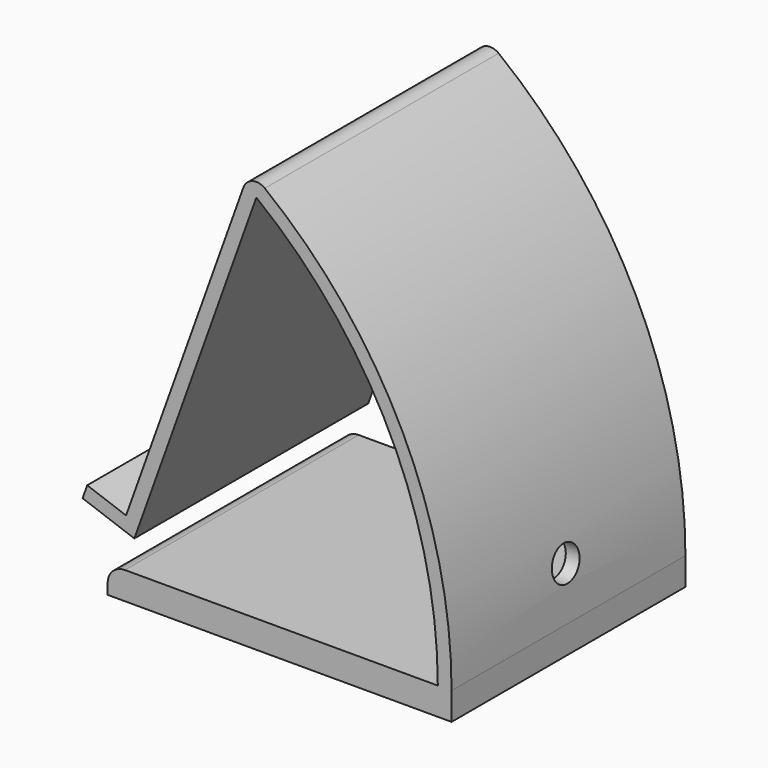
from build123d import *

# Parameters (mm, degrees)
F1_DEPTH = 85
F2_START = 22.5
F2_DEPTH = 40
F4_D     = 10
F4_DEPTH = 12
F4_START = 1.4311325
F4_TIP   = 3.0043030951


# Not quite as in the source:
# - a feature names something its author has since deleted; it is built from what else it names


with BuildPart() as f1:
    # F0 (on Front) → F1 (new body)
    with BuildSketch(Plane.XZ):
        with BuildLine():
            Line((-50, -4), (50, -4))
            Line((50, -4), (50, 4))
            Line((50, 4), (46, 4))
            Line((46, 4), (-45, 4))
            ThreePointArc((-45, 4), (-48.5355339059, 2.5355339059), (-50, -1))
            Line((-50, -1), (-50, -4))
        make_face()
        with BuildLine():
            Line((-6.7640438608, 111.7814914912), (-4.3106391095, 114.9407327175))
            ThreePointArc((-4.3106391095, 114.9407327175), (-7.8808210545, 115.6224300093), (-10.5289002901, 113.1327339074))
            Line((-10.5289002901, 113.1327339074), (-6.7640438608, 111.7814914912))
        make_face()
        with BuildLine():
            Line((46, 4), (50, 4))
            ThreePointArc((50, 4), (35.6938059368, 65.7606098099), (-4.3106391095, 114.9407327175))
            Line((-4.3106391095, 114.9407327175), (-6.7640438608, 111.7814914912))
            ThreePointArc((-6.7640438608, 111.7814914912), (32.1012011015, 64.0018629557), (46, 4))
        make_face()
        Polygon((-42.2341572851, 12.9540102238), (-6.7640438608, 111.7814914912), (-10.5289002901, 113.1327339074), (-44.6477712982, 18.0701090692), (-45.9990137144, 14.3052526399), align=None)
        Polygon((-45.9990137144, 14.3052526399), (-44.6477712982, 18.0701090692), (-55.9423405859, 22.1238363177), (-57.2935830021, 18.3589798884), align=None)
    extrude(amount=F1_DEPTH)

    # F0 (on Front) → F2 (cut)
    with BuildSketch(Plane.XZ.offset(F2_START)):
        Polygon((-45.9990137144, 14.3052526399), (-44.6477712982, 18.0701090692), (-55.9423405859, 22.1238363177), (-57.2935830021, 18.3589798884), align=None)
    extrude(amount=F2_DEPTH, mode=Mode.SUBTRACT)

    # F4
    # its depths count from where the whole tool has entered the part; down to there all is cleared
    with Locations(Plane.YZ.offset(50).offset(-F4_START)):
        with Locations((-42.5, 19)):
            Hole(F4_D / 2, depth=F4_DEPTH)
            with Locations((0, 0, -(F4_DEPTH + F4_TIP / 2))):  # 118° drill point
                Cone(0, F4_D / 2, F4_TIP, mode=Mode.SUBTRACT)


solid = f1.part
